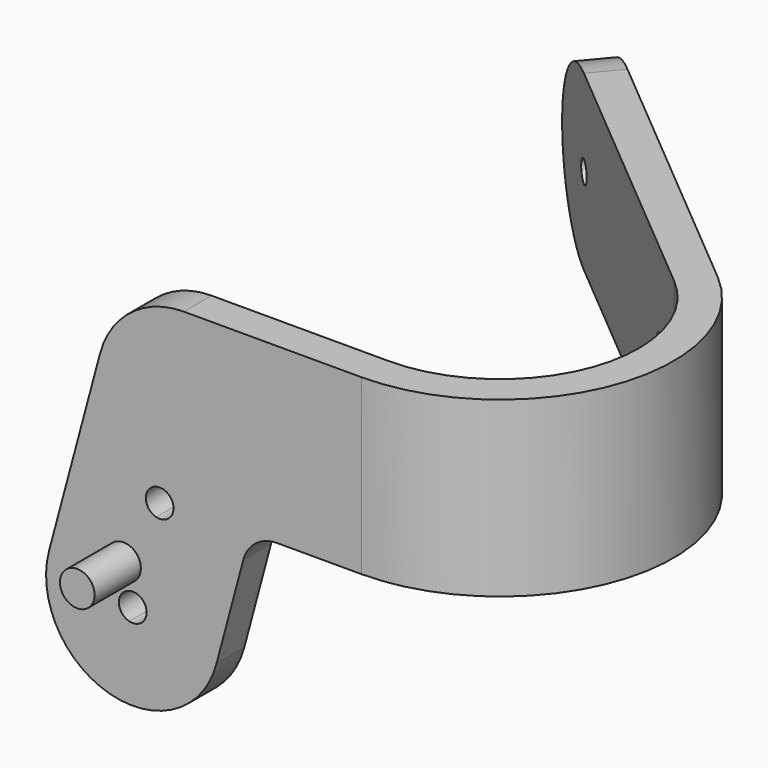
from build123d import *

# Parameters (mm, degrees)
F3_R      = 1.5
F4_DEPTH  = 5
F1_R      = 2.15
F5_DEPTH  = 25
F7_W      = 88.294127956
F7_H      = 15
F8_DEPTH  = 50
F0_W      = 181.6474571824
F0_H      = 159.0860895813
F9_DEPTH  = 39.5647038297
F10_R     = 0.95
F11_DEPTH = 5
F12_R     = 7.49999


# Not quite as in the source:
# - a fillet or chamfer is up to 0.001 mm smaller than in the source, because OpenCascade refuses the exact size


with BuildPart() as f4:
    # F3 (on offset) → F4 (new body)
    with BuildSketch(Plane.XZ.offset(1)):
        with Locations((0, -28.2000005245)):
            Circle(F3_R)
    extrude(amount=F4_DEPTH)


with BuildPart() as f5:
    # F1 (on Front) → F5 (new body)
    with BuildSketch(Plane.XZ):
        with BuildLine():
            ThreePointArc((-1.9411428383, -39.3081475268), (3.75, -38.5588943581), (7.2444436972, -34.0048466679))
            Line((7.2444436972, -34.0048466679), (9.5695999627, -25.3272453493))
            ThreePointArc((9.5695999627, -25.3272453493), (10.6410931546, -23.7236424637), (12.4673774416, -23.1037024846))
            Line((12.4673774416, -23.1037024846), (80.0844150527, -23.1037024846))
            ThreePointArc((80.0844150527, -23.1037024846), (87.5844150527, -15.6037024846), (80.0844150527, -8.1037024846))
            Line((80.0844150527, -8.1037024846), (49.0844150527, -8.1037024846))
            Line((49.0844150527, -8.1037024846), (19.777748386, -8.1037024846))
            Line((19.777748386, -8.1037024846), (4.4104440678, -8.1037024846))
            ThreePointArc((4.4104440678, -8.1037024846), (-0.1552666497, -9.6535524324), (-2.8339996293, -13.6625596463))
            Line((-2.8339996293, -13.6625596463), (-7.2444436972, -30.1225609914))
            ThreePointArc((-7.2444436972, -30.1225609914), (-6.4951905284, -35.8137038297), (-1.9411428383, -39.3081475268))
        make_face()
        with BuildLine():
            ThreePointArc((1.2, -32.0637038297), (0.7305137148, -33.015727838), (-0.3105828541, -33.2228148212))
            ThreePointArc((-0.3105828541, -33.2228148212), (-1.1591109915, -31.7531209756), (0.3105828541, -30.9045928381))
            ThreePointArc((0.3105828541, -30.9045928381), (0.9520240083, -31.3331901149), (1.2, -32.0637038297))
        make_face(mode=Mode.SUBTRACT)
        with BuildLine():
            ThreePointArc((3.5293714059, -23.3703713931), (3.0598851207, -24.3223954014), (2.0187885518, -24.5294823846))
            ThreePointArc((2.0187885518, -24.5294823846), (1.1702604144, -23.059788539), (2.63995426, -22.2112604015))
            ThreePointArc((2.63995426, -22.2112604015), (3.2813954143, -22.6398576783), (3.5293714059, -23.3703713931))
        make_face(mode=Mode.SUBTRACT)
        with Locations((54.0844150527, -15.6037024846)):
            Circle(F1_R, mode=Mode.SUBTRACT)
        with Locations((80.0844150527, -15.6037024846)):
            Circle(F1_R, mode=Mode.SUBTRACT)
    extrude(amount=-F5_DEPTH)

    # F7 (on offset) → F8 (join)
    with BuildSketch(Plane.XZ.offset(-25)):
        with Locations((17.6047375426, -15.6037024846)):
            Rectangle(F7_W, F7_H)
    extrude(amount=-F8_DEPTH)

    # F0 (on Top) → F9 (cut, through all)
    with BuildSketch(Plane.XY):
        with BuildLine():
            ThreePointArc((186.4293499082, 37.2767830718), (189.1206068421, 41.7118372377), (194.29723209, 41.3725432932))
            Line((194.29723209, 41.3725432932), (212.3185770643, 28.7538616935))
            Line((212.3185770643, 28.7538616935), (214.0393063734, 31.2113178264))
            Line((214.0393063734, 31.2113178264), (196.017961399, 43.8299994261))
            ThreePointArc((196.017961399, 43.8299994261), (187.7353610024, 44.3728697372), (183.4293499082, 37.2767830718))
            Line((183.4293499082, 37.2767830718), (183.4293499082, 8.5356936807))
            ThreePointArc((183.4293499082, 8.5356936807), (181.9648838142, 5.0001597747), (178.4293499082, 3.5356936807))
            Line((178.4293499082, 3.5356936807), (134.4964219123, 3.5356936807))
            Line((134.4964219123, 3.5356936807), (134.4964219123, 0.5356936807))
            Line((134.4964219123, 0.5356936807), (178.4293499082, 0.5356936807))
            ThreePointArc((178.4293499082, 0.5356936807), (184.0862041577, 2.8788394312), (186.4293499082, 8.5356936807))
            Line((186.4293499082, 8.5356936807), (186.4293499082, 37.2767830718))
        make_face()
        with Locations((32.1800746024, 51.0744024068)):
            Rectangle(F0_W, F0_H)
        with BuildLine():
            Line((19.777748386, 0), (0, 0))
            Line((0, 0), (-38.4993149038, 0))
            Line((-38.4993149038, 0), (-38.4993149038, 3))
            Line((-38.4993149038, 3), (0, 3))
            Line((0, 3), (19.777748386, 3))
            ThreePointArc((19.777748386, 3), (31.0540598354, 10.8957582801), (27.4911997022, 24.1925333174))
            Line((27.4911997022, 24.1925333174), (-2.0015113578, 48.9398562904))
            Line((-2.0015113578, 48.9398562904), (-0.0731485288, 51.2379896197))
            Line((-0.0731485288, 51.2379896197), (29.4195625313, 26.4906666468))
            ThreePointArc((29.4195625313, 26.4906666468), (33.8731376978, 9.8696978501), (19.777748386, 0))
        make_face(mode=Mode.SUBTRACT)
    extrude(amount=-F9_DEPTH, mode=Mode.SUBTRACT)

    # F10 (on face) → F11 (cut)
    with BuildSketch(Plane(origin=(25.1995615031, 30.0316679531, 0), x_dir=(-0.7660444431, 0.6427876097, 0), z_dir=(0.6427876097, 0.7660444431, 0))):
        with Locations((25.4911798968, -15.6037024846)):
            Circle(F10_R)
        with Locations((-0.5088201032, -15.6037024846)):
            Circle(F10_R)
    extrude(amount=-F11_DEPTH, mode=Mode.SUBTRACT)

    # F12 (radius 7.5 in the source; OpenCascade refuses exactly that, so slightly less here)
    f12_edges = [f5.edges().sort_by_distance(p)[0] for p in [
        (-1.03733, 50.088923, -8.103702),
        (-1.03733, 50.088923, -23.103702),
    ]]
    fillet(f12_edges, radius=F12_R)


solid = Compound([f4.part, f5.part])
